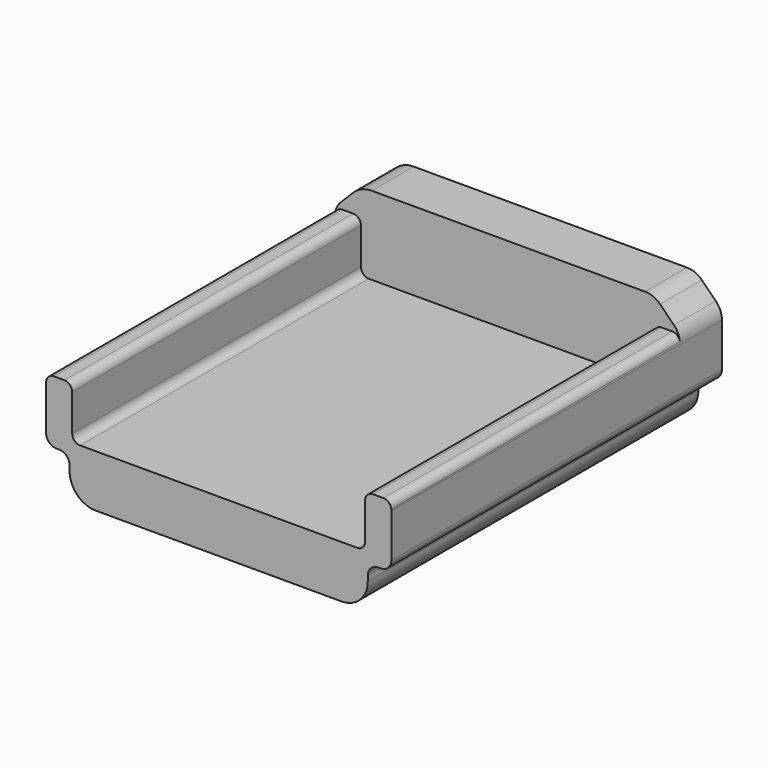
from build123d import *

# Parameters (mm, degrees)
F1_DEPTH  = 71
F3_DEPTH  = 8
F5_DEPTH  = 61
F6_SIZE   = 5
F7_SIZE   = 5
F8_R      = 4
F9_R      = 4
F10_R     = 4
F11_R     = 5
F12_W     = 5
F12_H     = 8
F13_DEPTH = 4.6
F14_W     = 5
F14_H     = 3
F15_DEPTH = 3
F16_W     = 5
F16_H     = 3
F17_DEPTH = 2
F19_DEPTH = 5
F20_R     = 2.75
F21_DEPTH = 3
F22_R     = 1.25
F23_DEPTH = 7


with BuildPart() as f1:
    # F0 (on Front) → F1 (new body)
    with BuildSketch(Plane.XZ):
        with BuildLine():
            Line((33, 12.5), (-33, 12.5))
            Line((-33, 12.5), (-33, -2.5))
            ThreePointArc((-33, -2.5), (-32.414214, -3.914214), (-31, -4.5))
            Line((-31, -4.5), (-30.5, -4.5))
            ThreePointArc((-30.5, -4.5), (-29.085786, -5.085786), (-28.5, -6.5))
            Line((-28.5, -6.5), (-28.5, -7.5))
            ThreePointArc((-28.5, -7.5), (-27.035534, -11.035534), (-23.5, -12.5))
            Line((-23.5, -12.5), (-13, -12.5))
            ThreePointArc((-13, -12.5), (-9.464466, -11.035534), (-8, -7.5))
            Line((-8, -7.5), (-8, -7))
            Line((-8, -7), (8, -7))
            Line((8, -7), (8, -7.5))
            ThreePointArc((8, -7.5), (9.464466, -11.035534), (13, -12.5))
            Line((13, -12.5), (23.5, -12.5))
            ThreePointArc((23.5, -12.5), (27.035534, -11.035534), (28.5, -7.5))
            Line((28.5, -7.5), (28.5, -6.5))
            ThreePointArc((28.5, -6.5), (29.085786, -5.085786), (30.5, -4.5))
            Line((30.5, -4.5), (31, -4.5))
            ThreePointArc((31, -4.5), (32.414214, -3.914214), (33, -2.5))
            Line((33, -2.5), (33, 12.5))
        make_face()
    extrude(amount=F1_DEPTH)

    # F2 (on face) → F3 (join)
    with BuildSketch(Plane.XZ.offset(71)):
        with BuildLine():
            Line((33, -2.317502), (33, 6))
            ThreePointArc((33, 6), (32.56066, 7.06066), (31.5, 7.5))
            Line((31.5, 7.5), (29.5, 7.5))
            ThreePointArc((29.5, 7.5), (28.43934, 7.06066), (28, 6))
            Line((28, 6), (28, -1))
            ThreePointArc((28, -1), (27.56066, -2.06066), (26.5, -2.5))
            Line((26.5, -2.5), (-26.5, -2.5))
            ThreePointArc((-26.5, -2.5), (-27.56066, -2.06066), (-28, -1))
            Line((-28, -1), (-28, 6))
            ThreePointArc((-28, 6), (-28.43934, 7.06066), (-29.5, 7.5))
            Line((-29.5, 7.5), (-31.5, 7.5))
            ThreePointArc((-31.5, 7.5), (-32.56066, 7.06066), (-33, 6))
            Line((-33, 6), (-33, -2.5))
            ThreePointArc((-33, -2.5), (-32.414214, -3.914214), (-31, -4.5))
            Line((-31, -4.5), (-30.5, -4.5))
            ThreePointArc((-30.5, -4.5), (-29.085786, -5.085786), (-28.5, -6.5))
            Line((-28.5, -6.5), (-28.5, -7.5))
            ThreePointArc((-28.5, -7.5), (-27.035534, -11.035534), (-23.5, -12.5))
            Line((-23.5, -12.5), (23.5, -12.5))
            ThreePointArc((23.5, -12.5), (27.035534, -11.035534), (28.5, -7.5))
            Line((28.5, -7.5), (28.5, -6.5))
            ThreePointArc((28.5, -6.5), (29.085786, -5.085786), (30.5, -4.5))
            Line((30.5, -4.5), (31, -4.5))
            ThreePointArc((31, -4.5), (32.414214, -3.914214), (33, -2.5))
            Line((33, -2.5), (33, -2.317502))
        make_face()
    extrude(amount=F3_DEPTH)

    # F4 (on face) → F5 (cut)
    with BuildSketch(Plane.XZ.offset(71)):
        with BuildLine():
            ThreePointArc((-29.5, 7.5), (-28.43934, 7.06066), (-28, 6))
            Line((-28, 6), (-28, -1))
            ThreePointArc((-28, -1), (-27.56066, -2.06066), (-26.5, -2.5))
            Line((-26.5, -2.5), (26.5, -2.5))
            ThreePointArc((26.5, -2.5), (27.56066, -2.06066), (28, -1))
            Line((28, -1), (28, 6))
            ThreePointArc((28, 6), (28.43934, 7.06066), (29.5, 7.5))
            Line((29.5, 7.5), (31.5, 7.5))
            ThreePointArc((31.5, 7.5), (32.56066, 7.06066), (33, 6))
            Line((33, 6), (33, 12.5))
            Line((33, 12.5), (-33, 12.5))
            Line((-33, 12.5), (-33, 6))
            ThreePointArc((-33, 6), (-32.56066, 7.06066), (-31.5, 7.5))
            Line((-31.5, 7.5), (-29.5, 7.5))
        make_face()
    extrude(amount=-F5_DEPTH, mode=Mode.SUBTRACT)

    # F6
    f6_edges = [f1.edges().sort_by_distance(p)[0] for p in [
        (-33, -5, 12.5),
    ]]
    chamfer(f6_edges, length=F6_SIZE)

    # F7
    f7_edges = [f1.edges().sort_by_distance(p)[0] for p in [
        (33, -5, 12.5),
    ]]
    chamfer(f7_edges, length=F7_SIZE)

    # F8
    f8_edges = [f1.edges().sort_by_distance(p)[0] for p in [
        (28, -5, 12.5),
    ]]
    fillet(f8_edges, radius=F8_R)

    # F9
    f9_edges = [f1.edges().sort_by_distance(p)[0] for p in [
        (33, -5, 7.5),
    ]]
    fillet(f9_edges, radius=F9_R)

    # F10
    f10_edges = [f1.edges().sort_by_distance(p)[0] for p in [
        (-33, -5, 7.5),
    ]]
    fillet(f10_edges, radius=F10_R)

    # F11
    f11_edges = [f1.edges().sort_by_distance(p)[0] for p in [
        (-28, -5, 12.5),
    ]]
    fillet(f11_edges, radius=F11_R)

    # F12 (on face) → F13 (join)
    with BuildSketch(Plane(origin=(0, 0, -7), x_dir=(1, 0, 0), z_dir=(0, 0, -1))):
        with Locations((-9, 55)):
            Rectangle(F12_W, F12_H)
        with Locations((9, 55)):
            Rectangle(F12_W, F12_H)
    extrude(amount=F13_DEPTH)

    # F14 (on face) → F15 (join)
    with BuildSketch(Plane(origin=(0, 0, -7), x_dir=(1, 0, 0), z_dir=(0, 0, -1))):
        with Locations((8, 34)):
            Rectangle(F14_W, F14_H)
        with Locations((8, 17.5)):
            Rectangle(F14_W, F14_H)
    extrude(amount=F15_DEPTH)

    # F16 (on face) → F17 (join)
    with BuildSketch(Plane(origin=(0, 0, -7), x_dir=(1, 0, 0), z_dir=(0, 0, -1))):
        with Locations((-8, 17.5)):
            Rectangle(F16_W, F16_H)
    extrude(amount=F17_DEPTH)

    # F18 (on face) → F19 (cut)
    with BuildSketch(Plane(origin=(0, 0, 0), x_dir=(-1, 0, 0), z_dir=(0, 1, 0))):
        with BuildLine():
            Line((8, -7), (-1.5, -7))
            Line((-1.5, -7), (-1.5, -12.5))
            Line((-1.5, -12.5), (13, -12.5))
            ThreePointArc((13, -12.5), (9.464466, -11.035534), (8, -7.5))
            Line((8, -7.5), (8, -7))
        make_face()
        with BuildLine():
            Line((28.5, -7), (8, -7))
            Line((8, -7), (8, -7.5))
            ThreePointArc((8, -7.5), (9.464466, -11.035534), (13, -12.5))
            Line((13, -12.5), (23.5, -12.5))
            ThreePointArc((23.5, -12.5), (27.035534, -11.035534), (28.5, -7.5))
            Line((28.5, -7.5), (28.5, -7))
        make_face()
    extrude(amount=-F19_DEPTH, mode=Mode.SUBTRACT)

    # F20 (on face) → F21 (cut)
    with BuildSketch(Plane(origin=(0, 0, -12.5), x_dir=(1, 0, 0), z_dir=(0, 0, -1))):
        with Locations((-17.75, 71)):
            Circle(F20_R)
        with Locations((17.75, 71)):
            Circle(F20_R)
        with Locations((17.75, 15.5)):
            Circle(F20_R)
        with Locations((-17.75, 15.5)):
            Circle(F20_R)
    extrude(amount=-F21_DEPTH, mode=Mode.SUBTRACT)

    # F22 (on face) → F23 (cut)
    with BuildSketch(Plane(origin=(0, 0, -12.5), x_dir=(1, 0, 0), z_dir=(0, 0, -1))):
        with Locations((-17.75, 71)):
            Circle(F22_R)
        with Locations((17.75, 71)):
            Circle(F22_R)
        with Locations((-17.75, 15.5)):
            Circle(F22_R)
        with Locations((17.75, 15.5)):
            Circle(F22_R)
    extrude(amount=-F23_DEPTH, mode=Mode.SUBTRACT)


solid = f1.part
